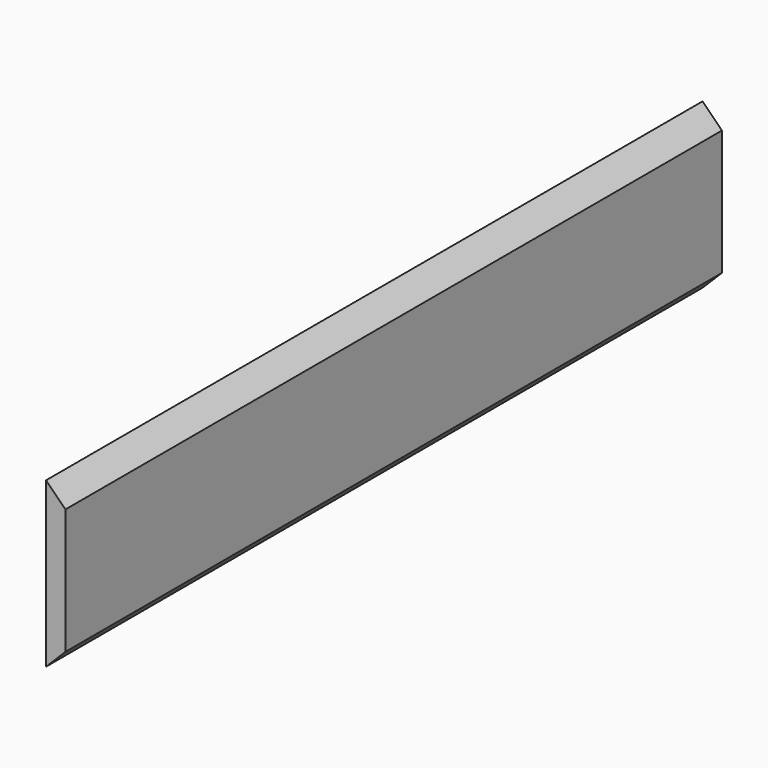
from build123d import *

# Parameters (mm, degrees)
F0_W     = 762
F0_H     = 152.4
F1_DEPTH = 17.99844
F2_SIZE  = 17.99843


# Not quite as in the source:
# - a fillet or chamfer is up to 0.001 mm smaller than in the source, because OpenCascade refuses the exact size


with BuildPart() as f1:
    # F0 (on Right) → F1 (new body)
    with BuildSketch(Plane.YZ):
        with Locations((-381, 76.2)):
            Rectangle(F0_W, F0_H)
    extrude(amount=F1_DEPTH)

    # F2 (size 17.99844 in the source; OpenCascade refuses exactly that, so slightly less here)
    f2_edges = [f1.edges().sort_by_distance(p)[0] for p in [
        (17.99844, -381, 152.4),
        (17.99844, -381, 0),
    ]]
    chamfer(f2_edges, length=F2_SIZE)


solid = f1.part
